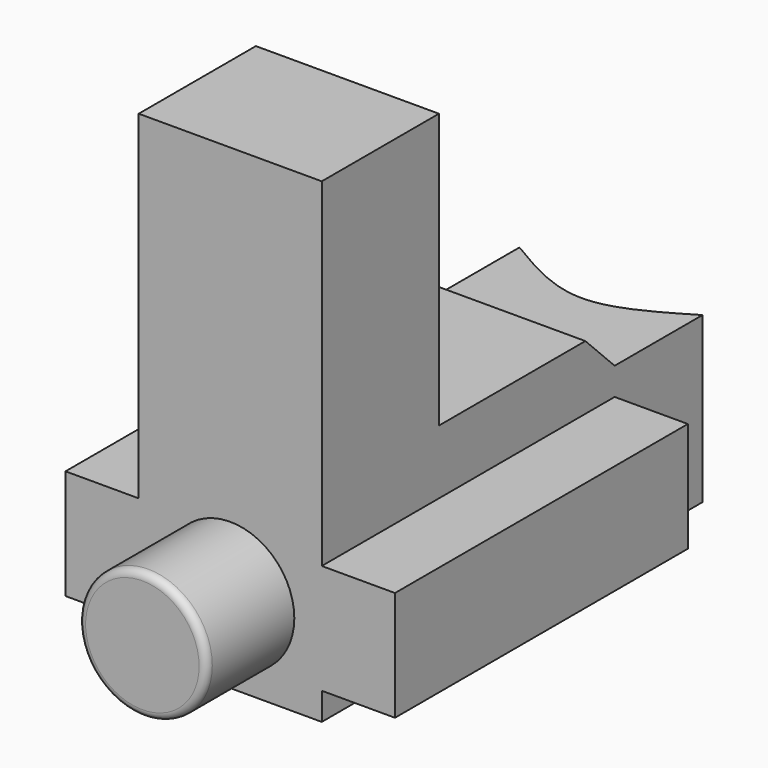
from build123d import *

# Parameters (mm, degrees)
F0_W     = 5
F0_H     = 7.5
F0_R     = 1.75
F0_H_2   = 1
F1_DEPTH = 4
F2_DEPTH = 3
F0_W_2   = 2
F0_H_3   = 3
F3_DEPTH = 10
F4_DEPTH = 13
F5_SIZE  = 0.99999
F7_DEPTH = 4.501
F8_R     = 0.2


# Not quite as in the source:
# - a fillet or chamfer is up to 0.001 mm smaller than in the source, because OpenCascade refuses the exact size


with BuildPart() as f1:
    # F0 (on Front) → F1 (new body)
    with BuildSketch(Plane.XZ):
        with Locations((2.5, 9.25)):
            Rectangle(F0_W, F0_H)
        Polygon((0, 0.75), (0, 0), (5, 0), (5, 0.75), (5, 3.75), (5, 4.5), (0, 4.5), (0, 3.75), align=None)
        with Locations((2.5, 2.25)):
            Circle(F0_R, mode=Mode.SUBTRACT)
        with Locations((2.5, 2.25)):
            Circle(F0_R)
        with Locations((2.5, 5)):
            Rectangle(F0_W, F0_H_2)
    extrude(amount=-F1_DEPTH)

    # F0 (on Front) → F2 (join)
    with BuildSketch(Plane.XZ):
        with Locations((2.5, 2.25)):
            Circle(F0_R)
    extrude(amount=F2_DEPTH)

    # F0 (on Front) → F3 (join)
    with BuildSketch(Plane.XZ):
        with Locations((6, 2.25)):
            Rectangle(F0_W_2, F0_H_3)
        with Locations((-1, 2.25)):
            Rectangle(F0_W_2, F0_H_3)
        with Locations((2.5, 5)):
            Rectangle(F0_W, F0_H_2)
        Polygon((0, 0.75), (0, 0), (5, 0), (5, 0.75), (5, 3.75), (5, 4.5), (0, 4.5), (0, 3.75), align=None)
        with Locations((2.5, 2.25)):
            Circle(F0_R, mode=Mode.SUBTRACT)
        with Locations((2.5, 2.25)):
            Circle(F0_R)
    extrude(amount=-F3_DEPTH)

    # F0 (on Front) → F4 (join)
    with BuildSketch(Plane.XZ):
        Polygon((0, 0.75), (0, 0), (5, 0), (5, 0.75), (5, 3.75), (5, 4.5), (0, 4.5), (0, 3.75), align=None)
        with Locations((2.5, 2.25)):
            Circle(F0_R, mode=Mode.SUBTRACT)
        with Locations((2.5, 2.25)):
            Circle(F0_R)
    extrude(amount=-F4_DEPTH)

    # F5 (size 1 in the source; OpenCascade refuses exactly that, so slightly less here)
    f5_edges = [f1.edges().sort_by_distance(p)[0] for p in [
        (2.5, 10, 5.5),
    ]]
    chamfer(f5_edges, length=F5_SIZE)

    # F6 (on face) → F7 (cut, through all)
    with BuildSketch(Plane.XY.offset(4.5)):
        with BuildLine():
            Line((5, 13), (2.5, 13))
            Line((2.5, 13), (2.5, 12))
            add(Edge.make_bspline(
                [(5, 13), (4.1666666667, 12.5), (3.3333333333, 12), (2.5, 12)],
                knots=[0, 0, 0, 0, 0.5, 0.5, 0.5, 0.5], degree=3))
        make_face()
        with BuildLine():
            Line((2.5, 12), (2.5, 13))
            Line((2.5, 13), (0, 13))
            add(Edge.make_bspline(
                [(2.5, 12), (1.6666666667, 12), (0.8333333333, 12.5), (0, 13)],
                knots=[0.5, 0.5, 0.5, 0.5, 1, 1, 1, 1], degree=3))
        make_face()
    extrude(amount=-F7_DEPTH, mode=Mode.SUBTRACT)

    # F8
    f8_edges = [f1.edges().sort_by_distance(p)[0] for p in [
        (0.75, -3, 2.25),
    ]]
    fillet(f8_edges, radius=F8_R)


solid = f1.part
